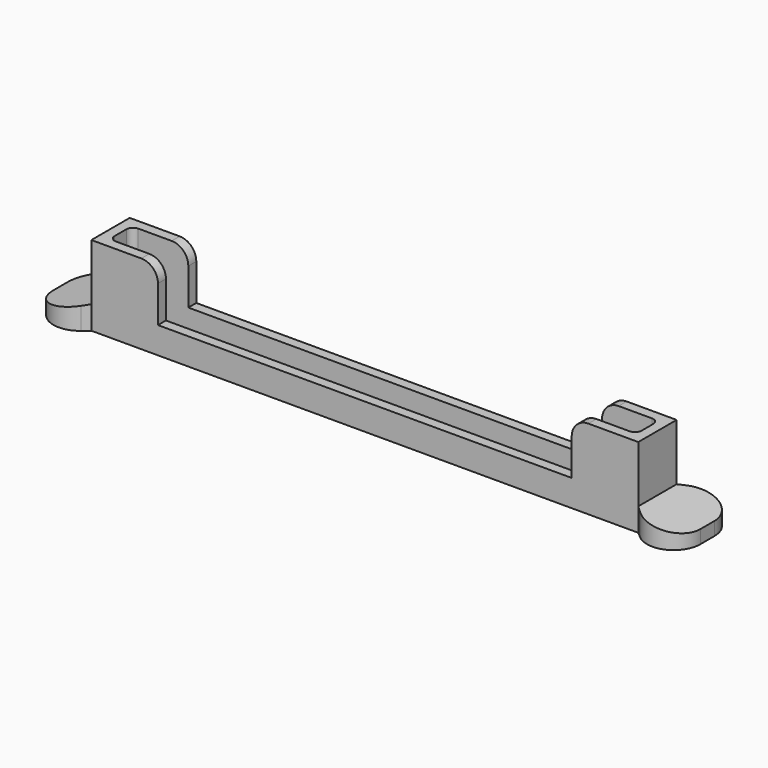
from build123d import *

# Parameters (mm, degrees)
F1_W         = 164.3
F1_H         = 14.4
F1_W_2       = 158.3
F1_H_2       = 8.4
F2_DEPTH     = 24
F3_T1_DEPTH  = 24
F5_DEPTH     = 4.35
F6_W         = 14.4
F6_H         = 7
F8_W         = 40
F8_H         = 4
F10_T1_DEPTH = 90.717403587
F11_W        = 124.3
F11_H        = 14.4
F12_DEPTH    = 16
F13_R        = 5


# Not quite as in the source:
# - a fillet or chamfer that OpenCascade refuses, or shapes differently, is made with other operations: its cross-section is extruded or revolved along the edge and cut away or added
# - a pattern or mirror of a feature is missing from the dataset's text; its kind, count and spacing are read off the source's solid


with BuildPart() as f2:
    # F1 (on Top) → F2 (new body)
    with BuildSketch(Plane.XY):
        Rectangle(F1_W, F1_H)
        Rectangle(F1_W_2, F1_H_2, mode=Mode.SUBTRACT)
    extrude(amount=F2_DEPTH)

    # F3: fillet of radius 2 on 4 edges, made by hand

    # F3_s2 → F3_t1 (join)
    with BuildSketch(Plane.XY):
        with BuildLine():
            ThreePointArc((79.1504, -2.1990343146), (78.5642135624, -3.6142135624), (77.1490343146, -4.2004))
            Line((77.1490343146, -4.2004), (77.1490343146, -4.4005365685))
            ThreePointArc((77.1490343146, -4.4005365685), (78.1495171573, -4.4001365685), (79.15, -4.4001365685))
            Line((79.15, -4.4001365685), (79.3501365685, -4.2))
            ThreePointArc((79.3501365685, -4.2), (79.3501365685, -3.1995171573), (79.3505365685, -2.1990343146))
            Line((79.3505365685, -2.1990343146), (79.1504, -2.1990343146))
        make_face()
        with BuildLine():
            ThreePointArc((79.1504, 2.1990343146), (78.5642135624, 3.6142135624), (77.1490343146, 4.2004))
            Line((77.1490343146, 4.2004), (77.1490343146, 4.4005365685))
            ThreePointArc((77.1490343146, 4.4005365685), (78.1495171573, 4.4001365685), (79.15, 4.4001365685))
            Line((79.15, 4.4001365685), (79.3501365685, 4.2))
            ThreePointArc((79.3501365685, 4.2), (79.3501365685, 3.1995171573), (79.3505365685, 2.1990343146))
            Line((79.3505365685, 2.1990343146), (79.1504, 2.1990343146))
        make_face()
        with BuildLine():
            ThreePointArc((-77.1490343146, -4.2004), (-78.5642135624, -3.6142135624), (-79.1504, -2.1990343146))
            Line((-79.1504, -2.1990343146), (-79.3505365685, -2.1990343146))
            ThreePointArc((-79.3505365685, -2.1990343146), (-79.3501365685, -3.1995171573), (-79.3501365685, -4.2))
            Line((-79.3501365685, -4.2), (-79.15, -4.4001365685))
            ThreePointArc((-79.15, -4.4001365685), (-78.1495171573, -4.4001365685), (-77.1490343146, -4.4005365685))
            Line((-77.1490343146, -4.4005365685), (-77.1490343146, -4.2004))
        make_face()
        with BuildLine():
            ThreePointArc((-79.1504, 2.1990343146), (-78.5642135624, 3.6142135624), (-77.1490343146, 4.2004))
            Line((-77.1490343146, 4.2004), (-77.1490343146, 4.4005365685))
            ThreePointArc((-77.1490343146, 4.4005365685), (-78.1495171573, 4.4001365685), (-79.15, 4.4001365685))
            Line((-79.15, 4.4001365685), (-79.3501365685, 4.2))
            ThreePointArc((-79.3501365685, 4.2), (-79.3501365685, 3.1995171573), (-79.3505365685, 2.1990343146))
            Line((-79.3505365685, 2.1990343146), (-79.1504, 2.1990343146))
        make_face()
    extrude(amount=F3_T1_DEPTH)

    # F4 (on Front) → F5 (join, symmetric)
    with BuildSketch(Plane.XZ):
        with BuildLine():
            ThreePointArc((79.15, 8.75), (76.8068542495, 3.0931457505), (71.15, 0.75))
            Line((71.15, 0.75), (71.15, 0))
            Line((71.15, 0), (82.15, 0))
            Line((82.15, 0), (82.15, 8.75))
            Line((82.15, 8.75), (79.15, 8.75))
        make_face()
    f5 = extrude(amount=F5_DEPTH, both=True)

    # F5_copies: F5 across plane
    add(f5.mirror(Plane(origin=(0, 0, 0), x_dir=(0, 0, -1), z_dir=(-1, 0, 0))))

    # F6 (on face) → F9 section 0
    with BuildSketch(Plane(origin=(-82.15, 0, 0), x_dir=(0, -1, 0), z_dir=(-1, 0, 0))):
        with Locations((0, 3.5)):
            Rectangle(F6_W, F6_H)
    # F8 (on offset) → F9 section 1
    with BuildSketch(Plane(origin=(-97.15, 0, 0), x_dir=(0, -1, 0), z_dir=(-1, 0, 0))):
        with Locations((0, 2)):
            Rectangle(F8_W, F8_H)
    f9 = loft()

    # F9_copies: F9 across plane
    add(f9.mirror(Plane(origin=(0, 0, 0), x_dir=(0, 0, 1), z_dir=(1, 0, 0))))

    # F10: fillet of radius 8 on 4 edges, made by hand

    # F10_s2 → F10_t1 (cut)
    with BuildSketch(Plane.XY.offset(-43.3587017935)):
        with BuildLine():
            ThreePointArc((-97.15, 2.6565192826), (-92.500848152, 9.9209405715), (-83.9570458344, 8.7420124454))
            Line((-83.9570458344, 8.7420124454), (-97.15, 20))
            Line((-97.15, 20), (-97.15, 2.6565192826))
        make_face()
        with BuildLine():
            ThreePointArc((-83.9570458344, -8.7420124454), (-92.500848152, -9.9209405715), (-97.15, -2.6565192826))
            Line((-97.15, -2.6565192826), (-97.15, -20))
            Line((-97.15, -20), (-83.9570458344, -8.7420124454))
        make_face()
        with BuildLine():
            ThreePointArc((83.9570458344, -8.7420124454), (92.500848152, -9.9209405715), (97.15, -2.6565192826))
            Line((97.15, -2.6565192826), (97.15, -20))
            Line((97.15, -20), (83.9570458344, -8.7420124454))
        make_face()
        with BuildLine():
            ThreePointArc((97.15, 2.6565192826), (92.500848152, 9.9209405715), (83.9570458344, 8.7420124454))
            Line((83.9570458344, 8.7420124454), (97.15, 20))
            Line((97.15, 20), (97.15, 2.6565192826))
        make_face()
    extrude(amount=F10_T1_DEPTH, mode=Mode.SUBTRACT)

    # F11 (on face) → F12 (cut)
    with BuildSketch(Plane.XY.offset(24)):
        Rectangle(F11_W, F11_H)
    extrude(amount=-F12_DEPTH, mode=Mode.SUBTRACT)

    # F13
    f13_edges = [f2.edges().sort_by_distance(p)[0] for p in [
        (-62.15, 5.7, 24),
        (-62.15, -5.7, 24),
        (62.15, 5.7, 24),
        (62.15, -5.7, 24),
    ]]
    fillet(f13_edges, radius=F13_R)


solid = f2.part
